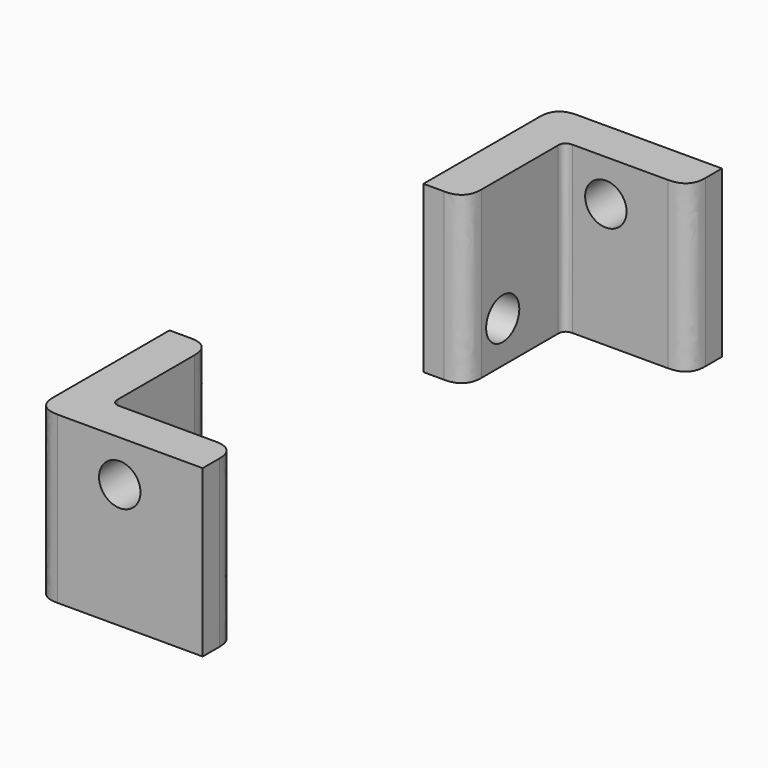
from build123d import *

# Parameters (mm, degrees)
F1_DEPTH       = 25.4
F3_R           = 3.175
F4_DEPTH       = 6.35
F2_R           = 3.175
F5_DEPTH       = 6.35
F7_DEPTH       = 25.4
F8_R           = 3.175
F9_DEPTH       = 6.35
F10_R          = 3.175
F11_DEPTH      = 6.35
F12_T1_DEPTH   = 41.275
F12_2_T1_DEPTH = 41.275
F13_T1_DEPTH   = 41.275
F13_2_T1_DEPTH = 41.275
F14_T1_DEPTH   = 25.4
F14_2_T1_DEPTH = 25.4


# Not quite as in the source:
# - a fillet or chamfer that OpenCascade refuses, or shapes differently, is made with other operations: its cross-section is extruded or revolved along the edge and cut away or added


with BuildPart() as f1:
    # F0 (on Top) → F1 (new body)
    with BuildSketch(Plane.XY):
        Polygon((-32.7995864883, 0), (-39.1495864883, 0), (-39.1495864883, -25.4), (-13.7495864883, -25.4), (-13.7495864883, -19.05), (-32.7995864883, -19.05), align=None)
    extrude(amount=F1_DEPTH)

    # F3 (on face) → F4 (cut)
    with BuildSketch(Plane(origin=(0, -19.05, 0), x_dir=(-1, 0, 0), z_dir=(0, 1, 0))):
        with Locations((26.4495864883, 19.05)):
            Circle(F3_R)
    extrude(amount=-F4_DEPTH, mode=Mode.SUBTRACT)

    # F2 (on face) → F5 (cut)
    with BuildSketch(Plane.YZ.offset(-32.7995864883)):
        with Locations((-7.239, 6.35)):
            Circle(F2_R)
    extrude(amount=-F5_DEPTH, mode=Mode.SUBTRACT)

    # F12#2: fillet of radius 3.175 on 2 edges, made by hand

    # F12_2_s2 → F12_2_t1 (cut)
    with BuildSketch(Plane.XY.offset(-7.9375)):
        with BuildLine():
            add(Edge.make_bspline(
                [(-35.9745864883, 0), (-32.7995864883, 0), (-32.7995864883, -3.175)],
                knots=[0, 0, 0, 1, 1, 1], degree=2, weights=[1, 1, 1]))
            Line((-32.7995864883, -3.175), (-32.7995864883, 0))
            Line((-32.7995864883, 0), (-35.9745864883, 0))
        make_face()
        with BuildLine():
            add(Edge.make_bspline(
                [(-16.9245864883, -19.05), (-13.7495864883, -19.05), (-13.7495864883, -22.225)],
                knots=[0, 0, 0, 1, 1, 1], degree=2, weights=[1, 1, 1]))
            Line((-13.7495864883, -22.225), (-13.7495864883, -19.05))
            Line((-13.7495864883, -19.05), (-16.9245864883, -19.05))
        make_face()
    extrude(amount=F12_2_T1_DEPTH, mode=Mode.SUBTRACT)

    # F13: fillet of radius 3.175 on 1 edges, made by hand

    # F13_s2 → F13_t1 (cut)
    with BuildSketch(Plane.XY.offset(-7.9375)):
        with BuildLine():
            add(Edge.make_bspline(
                [(-39.1495864883, -22.225), (-39.1495864883, -25.4), (-35.9745864883, -25.4)],
                knots=[0, 0, 0, 1, 1, 1], degree=2, weights=[1, 1, 1]))
            Line((-35.9745864883, -25.4), (-39.1495864883, -25.4))
            Line((-39.1495864883, -25.4), (-39.1495864883, -22.225))
        make_face()
    extrude(amount=F13_T1_DEPTH, mode=Mode.SUBTRACT)

    # F14#2: fillet of radius 1.27 on 1 edges, made by hand

    # F14_2_s2 → F14_2_t1 (join)
    with BuildSketch(Plane.XY):
        with BuildLine():
            add(Edge.make_bspline(
                [(-32.7995864883, -17.78), (-32.7995864883, -19.05), (-31.5295864883, -19.05)],
                knots=[0, 0, 0, 1, 1, 1], degree=2, weights=[1, 1, 1]))
            Line((-31.5295864883, -19.05), (-32.7995864883, -19.05))
            Line((-32.7995864883, -19.05), (-32.7995864883, -17.78))
        make_face()
    extrude(amount=F14_2_T1_DEPTH)


with BuildPart() as f7:
    # F6 (on Top) → F7 (new body)
    with BuildSketch(Plane.XY):
        Polygon((-39.1495864883, 48.6232675612), (-32.7995864883, 48.6232675612), (-32.7995864883, 67.6732675612), (-13.7495864883, 67.6732675612), (-13.7495864883, 74.0232675612), (-39.1495864883, 74.0232675612), align=None)
    extrude(amount=F7_DEPTH)

    # F8 (on face) → F9 (cut)
    with BuildSketch(Plane.YZ.offset(-32.7995864883)):
        with Locations((55.8622675612, 6.35)):
            Circle(F8_R)
    extrude(amount=-F9_DEPTH, mode=Mode.SUBTRACT)

    # F10 (on face) → F11 (cut)
    with BuildSketch(Plane.XZ.offset(-67.6732675612)):
        with Locations((-26.4495864883, 19.05)):
            Circle(F10_R)
    extrude(amount=-F11_DEPTH, mode=Mode.SUBTRACT)

    # F12: fillet of radius 3.175 on 2 edges, made by hand

    # F12_s2 → F12_t1 (cut)
    with BuildSketch(Plane.XY.offset(-7.9375)):
        with BuildLine():
            add(Edge.make_bspline(
                [(-13.7495864883, 70.8482675612), (-13.7495864883, 67.6732675612), (-16.9245864883, 67.6732675612)],
                knots=[0, 0, 0, 1, 1, 1], degree=2, weights=[1, 1, 1]))
            Line((-16.9245864883, 67.6732675612), (-13.7495864883, 67.6732675612))
            Line((-13.7495864883, 67.6732675612), (-13.7495864883, 70.8482675612))
        make_face()
        with BuildLine():
            add(Edge.make_bspline(
                [(-35.9745864883, 48.6232675612), (-32.7995864883, 48.6232675612), (-32.7995864883, 51.7982675612)],
                knots=[0, 0, 0, 1, 1, 1], degree=2, weights=[1, 1, 1]))
            Line((-32.7995864883, 51.7982675612), (-32.7995864883, 48.6232675612))
            Line((-32.7995864883, 48.6232675612), (-35.9745864883, 48.6232675612))
        make_face()
    extrude(amount=F12_T1_DEPTH, mode=Mode.SUBTRACT)

    # F13#2: fillet of radius 3.175 on 1 edges, made by hand

    # F13_2_s2 → F13_2_t1 (cut)
    with BuildSketch(Plane.XY.offset(-7.9375)):
        with BuildLine():
            add(Edge.make_bspline(
                [(-39.1495864883, 70.8482675612), (-39.1495864883, 74.0232675612), (-35.9745864883, 74.0232675612)],
                knots=[0, 0, 0, 1, 1, 1], degree=2, weights=[1, 1, 1]))
            Line((-35.9745864883, 74.0232675612), (-39.1495864883, 74.0232675612))
            Line((-39.1495864883, 74.0232675612), (-39.1495864883, 70.8482675612))
        make_face()
    extrude(amount=F13_2_T1_DEPTH, mode=Mode.SUBTRACT)

    # F14: fillet of radius 1.27 on 1 edges, made by hand

    # F14_s2 → F14_t1 (join)
    with BuildSketch(Plane.XY):
        with BuildLine():
            add(Edge.make_bspline(
                [(-31.5295864883, 67.6732675612), (-32.7995864883, 67.6732675612), (-32.7995864883, 66.4032675612)],
                knots=[0, 0, 0, 1, 1, 1], degree=2, weights=[1, 1, 1]))
            Line((-32.7995864883, 66.4032675612), (-32.7995864883, 67.6732675612))
            Line((-32.7995864883, 67.6732675612), (-31.5295864883, 67.6732675612))
        make_face()
    extrude(amount=F14_T1_DEPTH)


solid = Compound([f1.part, f7.part])
